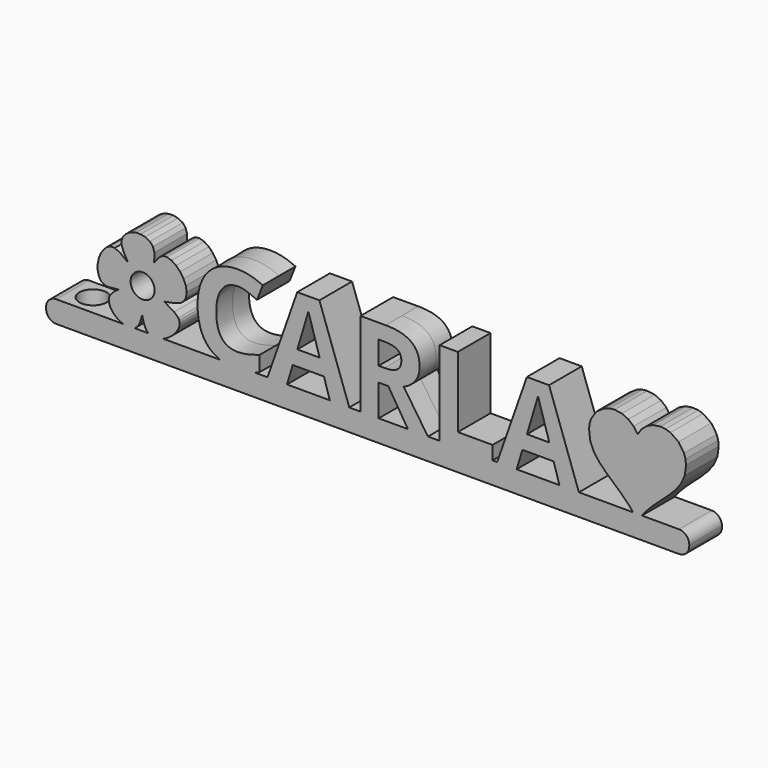
from build123d import *

# Parameters (mm, degrees)
F0_R         = 1.7660260944
F0_TEXT_SIZE = 17.6180462627
F1_DEPTH     = 3
F2_W         = 87
F2_H         = 6
F3_DEPTH     = 0.2
F4_DEPTH     = 3
F5_W         = 6
F5_H         = 3.2
F6_DEPTH     = 7.5
F7_R         = 1.5
F8_R         = 2
F9_DEPTH     = 4
F10_R        = 1.5


# Not quite as in the source:
# - Text() gives the source's letters only with a copy of the font that has no kerning and outlines rounded to 1/6400 em; it was checked with that copy


with BuildPart() as f1:
    # F0 (on Front) → F1 (new body, symmetric)
    with BuildSketch(Plane.XZ):
        Polygon((-9.8962181259, -0.0299609487), (-9.3093152472, 0.0995427735), (-8.5310452338, 0.4643787281), (-7.7886221935, 1.0156229815), (-7.1753136859, 1.6703047867), (-6.7844076966, 2.345448762), (-6.6844409889, 2.697736103), (-6.6652413988, 3.0240118702), (-6.7312263226, 3.3305926174), (-6.8868132072, 3.6238062576), (-7.4844896445, 4.1953846804), (-8.4936258745, 4.789299945), (-8.9274018823, 5.0567831788), (-8.4181052429, 5.1580766137), (-7.3131137554, 5.3695361907), (-6.5480905692, 5.6521941874), (-6.0523445823, 6.043851435), (-5.7552051187, 6.5823041299), (-5.6420905942, 7.3346827833), (-5.7751165223, 8.1369112107), (-6.1089634595, 8.9328581362), (-6.5983028952, 9.6663968681), (-7.1978267956, 10.281407439), (-7.8622157172, 10.7217585729), (-8.546147975, 10.9313258196), (-8.8812811082, 10.9320270148), (-9.2043064176, 10.8539824368), (-9.6469000392, 10.5612860557), (-10.1400767255, 9.9810366231), (-10.4508130024, 9.5801644376), (-10.4068223535, 10.0271686751), (-10.3916193646, 10.9311557532), (-10.598433195, 11.6324207168), (-11.0363252865, 12.1480644274), (-11.7143548393, 12.4951945719), (-12.3982545289, 12.6383143795), (-13.0712303381, 12.6247535348), (-13.7032208938, 12.4733707309), (-14.2641853, 12.2030313855), (-14.7240621838, 11.8325941916), (-15.0528129411, 11.3809291004), (-15.2203761991, 10.8668948051), (-15.1967042361, 10.3093544817), (-14.8286469794, 9.4077545862), (-14.3529716358, 8.5454741101), (-14.2906102139, 8.4004774316), (-14.4811582303, 8.5293860258), (-15.3946726039, 9.2300894295), (-16.21802192, 9.6332437342), (-16.8030362894, 9.634121823), (-17.3568401554, 9.3699870508), (-17.8525159958, 8.8932532172), (-18.2631576982, 8.2563454299), (-18.5618432066, 7.5116797807), (-18.7216618753, 6.7116836696), (-18.7156984739, 5.9087754295), (-18.5170445979, 5.1553756349), (-18.2008868091, 4.6439944488), (-17.7512302174, 4.3560670179), (-17.1086136552, 4.2712956407), (-16.2135760559, 4.3694053341), (-15.7044514474, 4.4302814773), (-15.6696932647, 4.4000047008), (-15.7790195709, 4.3290260096), (-16.1651405309, 4.0708069691), (-16.5523139664, 3.7127982689), (-16.8671052824, 3.3322639471), (-17.0360798838, 3.0064680418), (-17.0831036318, 2.6043628391), (-17.0239245605, 2.1921008316), (-16.867618816, 1.7819255621), (-16.6232807801, 1.3860941234), (-16.3000002503, 1.0168545414), (-15.9068693162, 0.6864593752), (-15.4529754831, 0.4071521172), (-14.9474063577, 0.1911989779), (-14.4397479673, 0.0570083052), (-13.9840845603, 0.0188926715), (-13.5797273957, 0.0772799851), (-13.2259605822, 0.2326232662), (-12.9220907946, 0.485341356), (-12.6674066752, 0.8358849825), (-12.4612081239, 1.2846821047), (-12.3027905578, 1.8321743328), (-12.1879723822, 2.2557758958), (-12.1309056827, 2.0998483864), (-12.0112204133, 1.5291342486), (-11.8237778137, 0.9902805659), (-11.5954117235, 0.5466869075), (-11.3529559319, 0.2617414835), (-10.9521058183, 0.053843468), (-10.4551700276, -0.0442881949), align=None)
        with Locations((-12.1185852993, 6.0541479067)):
            Circle(F0_R, mode=Mode.SUBTRACT)
        Polygon((58.3035863837, 12.4433699982), (57.2425663837, 12.5970599982), (56.4839563837, 12.5204799982), (55.7771563837, 12.3008699982), (54.5798163837, 11.4933499982), (53.7721963837, 10.2961199982), (53.5525463837, 9.5893599982), (53.4759563837, 8.8307599982), (53.6644763837, 7.3860999982), (54.1852163837, 6.1597099982), (54.9709663837, 5.0814099982), (55.9544963837, 4.0810299982), (58.2513463837, 2.0250499982), (59.4359363837, 0.8247399982), (60.5589263837, -0.5860800018), (60.6032063837, -0.6500000018), (60.6462363837, -0.5851400018), (61.7241463837, 0.8234499982), (62.8874463837, 2.0333299982), (65.1911163837, 4.1212499982), (66.1919063837, 5.1327499982), (66.9969063837, 6.2116199982), (67.5332963837, 7.4226699982), (67.7282763837, 8.8307599982), (67.6516963837, 9.5893599982), (67.4320863837, 10.2961199982), (66.6245663837, 11.4933499982), (65.4273363837, 12.3008699982), (64.7205663837, 12.5204799982), (63.9619763837, 12.5970599982), (62.9009563837, 12.4433699982), (61.9598863837, 12.0123599982), (61.1799363837, 11.3491699982), (60.6022663837, 10.4989199982), (60.0246063837, 11.3491699982), (59.2446563837, 12.0123599982), align=None)
        with Locations((-5.0661823743, 0)):
            Text('CARLA', F0_TEXT_SIZE, font='Open Sans', font_style=FontStyle.BOLD, text_align=(TextAlign.LEFT, TextAlign.BOTTOM))
    extrude(amount=F1_DEPTH, both=True)



with BuildPart() as f3:
    # F2 (on Top) → F3 (new body)
    with BuildSketch(Plane.XY):
        with Locations((24.7, 0)):
            Rectangle(F2_W, F2_H)
    extrude(amount=F3_DEPTH)


with BuildPart() as f4:
    # F4 (new): a face of the model
    f4_faces = [f3.part.faces().sort_by_distance(p)[0] for p in [
        (24.7, 0, 0),
    ]]
    extrude(f4_faces, amount=F4_DEPTH)


with BuildPart() as f1_1:
    add(f1.part)

    add(f3.part)  # F6 merges F3

    add(f4.part)  # F6 merges F4
    # F5 (on face) → F6 (join)
    with BuildSketch(Plane(origin=(-18.8, 0, 0), x_dir=(0, -1, 0), z_dir=(-1, 0, 0))):
        with Locations((0, -1.4)):
            Rectangle(F5_W, F5_H)
    extrude(amount=F6_DEPTH)

    # F7
    f7_edges = [f1_1.edges().sort_by_distance(p)[0] for p in [
        (-26.3, 0, -3),
        (-26.3, 0, 0.2),
        (68.2, 0, -3),
    ]]
    fillet(f7_edges, radius=F7_R)

    # F8 (on face) → F9 (cut)
    with BuildSketch(Plane.XY.offset(0.2)):
        with Locations((-21.8, 0)):
            Circle(F8_R)
    extrude(amount=-F9_DEPTH, mode=Mode.SUBTRACT)

    # F10
    f10_edges = [f1_1.edges().sort_by_distance(p)[0] for p in [
        (68.2, 0, 0.2),
    ]]
    fillet(f10_edges, radius=F10_R)


solid = f1_1.part
